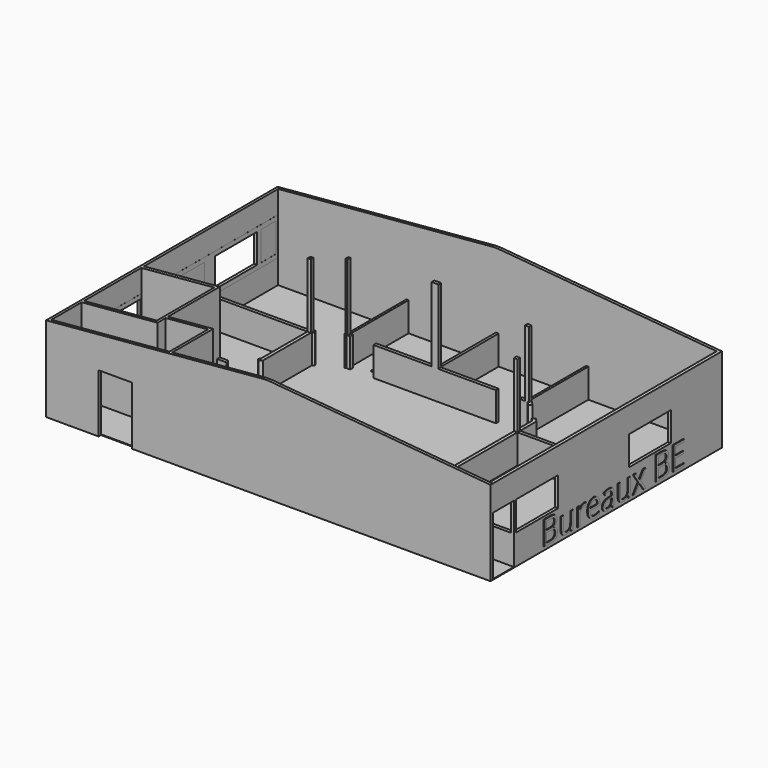
from build123d import *

# Parameters (mm, degrees)
F0_W            = 15040
F0_H            = 9720
F1_DEPTH        = 25
F2_W            = 15240
F2_H            = 9920
F2_W_2          = 100
F2_H_2          = 2105
F3_DEPTH        = 3550
F3_DEPTH_BACK   = 25
F4_W            = 1800
F4_H            = 1000
F5_DEPTH        = 100
F6_W            = 1800
F6_H            = 1000
F7_DEPTH        = 100
F8_W            = 1150
F8_H            = 2000
F9_DEPTH        = 100
F10_W           = 800
F10_H           = 2000
F11_DEPTH       = 100
F13_DEPTH       = 9920.001
F14_W           = 900
F14_H           = 2000
F15_DEPTH       = 100
F16_W           = 115
F16_H           = 115
F16_W_2         = 75
F16_W_3         = 126.4718625761
F16_W_4         = 85
F16_H_2         = 2500
F17_DEPTH       = 2550
F19_DEPTH       = 1
F20_W           = 1150
F20_H           = 1995.2939233818
F21_DEPTH       = 1
F22_W           = 1557.891368866
F22_H           = 1000
F22_W_2         = 1800
F22_W_3         = 1859.8644733429
F23_DEPTH       = 1
F24_W           = 1557.891368866
F24_H           = 1000
F24_W_2         = 1800
F24_W_3         = 1859.8644733429
F25_DEPTH       = 1
F26_W           = 8319
F26_H           = 2928.7534618515
F26_W_2         = 1800
F26_H_2         = 1000
F26_W_3         = 2364.8843765259
F26_W_4         = 644.2222595215
F27_DEPTH       = 1
F28_W           = 8319
F28_H           = 1300
F28_W_2         = 1800
F28_H_2         = 1000
F28_W_3         = 2364.8843765259
F28_W_4         = 644.2222595215
F29_DEPTH       = 1
F30_W           = 1150
F30_H           = 2000
F31_DEPTH       = 1
F32_W           = 800
F32_H           = 115
F33_DEPTH       = 1000
F34_TEXT_SIZE   = 952.5378545125
F34_TEXT_SIZE_2 = 810.1748095618
F35_DEPTH       = 25
F36_TEXT_SIZE   = 1144.444435421
F37_DEPTH       = 25


# Not quite as in the source:
# - Text() gives the source's letters only with a copy of the font that has no kerning and outlines rounded to 1/6400 em; it was checked with that copy


with BuildPart() as f1:
    # F0 (on Top) → F1 (new body)
    with BuildSketch(Plane.XY):
        with Locations((-7520, 4860)):
            Rectangle(F0_W, F0_H)
    extrude(amount=F1_DEPTH)

    # F2 (on face) → F3 (join, two sides)
    with BuildSketch(Plane.XY.offset(25)) as f3_sk:
        with Locations((-7520, 4860)):
            Rectangle(F2_W, F2_H)
        Polygon((-15040, 0), (-15040, 1300), (-15040, 1400), (-15040, 3855), (-15040, 3970), (-15040, 6605), (-15040, 6720), (-15040, 9720), (-10640, 9720), (-10565, 9720), (-7565, 9720), (-7475, 9720), (-4475, 9720), (-4400, 9720), (0, 9720), (0, 5670), (0, 5555), (0, 1015), (0, 900), (0, 0), (-10890, 0), (-10990, 0), align=None, mode=Mode.SUBTRACT)
        Polygon((-15040, 1400), (-15040, 1300), (-12440, 1300), (-12440, 1650), (-10990, 1650), (-10990, 0), (-10890, 0), (-10890, 1750), (-12440, 1750), (-12540, 1750), (-12540, 1400), align=None)
        with Locations((-12490, 2802.5)):
            Rectangle(F2_W_2, F2_H_2)
        Polygon((-15040, 3970), (-15040, 3855), (-12540, 3855), (-12440, 3855), (-12117.9646455628, 3855), (-11425, 4547.9646455628), (-11425, 6652.3336148652), (-10610.2005067573, 7105), (-4396.1626970968, 7105), (-3615, 6323.8373029032), (-3615, 4846.8259293999), (-3615, 2035.0966799188), (-2479.9033200812, 900), (0, 900), (0, 1015), (-2432.2687604083, 1015), (-3500, 2082.7312395917), (-3500, 5555), (0, 5555), (0, 5670), (-3500, 5670), (-3500, 6371.4718625761), (-4348.5281374239, 7220), (-4400, 7220), (-4400, 9720), (-4475, 9720), (-4475, 7220), (-7475, 7220), (-7475, 9720), (-7565, 9720), (-7565, 7220), (-10565, 7220), (-10565, 9720), (-10640, 9720), (-10640, 7220), (-11540, 6720), (-15040, 6720), (-15040, 6605), (-11540, 6605), (-11540, 4595.5992052357), (-12165.5992052357, 3970), align=None)
    extrude(amount=F3_DEPTH)
    extrude(f3_sk.sketch, amount=-F3_DEPTH_BACK)

    # F4 (on face) → F5 (cut, through all)
    with BuildSketch(Plane.YZ.offset(100)):
        with Locations((1900, 1525)):
            Rectangle(F4_W, F4_H)
        with Locations((6730, 1525)):
            Rectangle(F4_W, F4_H)
    extrude(amount=-F5_DEPTH, mode=Mode.SUBTRACT)

    # F6 (on face) → F7 (cut, through all)
    with BuildSketch(Plane(origin=(-15140, 0, 0), x_dir=(0, -1, 0), z_dir=(-1, 0, 0))):
        with Locations((-7920, 1500)):
            Rectangle(F6_W, F6_H)
        with Locations((-2910, 1500)):
            Rectangle(F6_W, F6_H)
    extrude(amount=-F7_DEPTH, mode=Mode.SUBTRACT)

    # F8 (on face) → F9 (cut, through all)
    with BuildSketch(Plane.XZ.offset(100)):
        with Locations((-12765, 1000)):
            Rectangle(F8_W, F8_H)
    extrude(amount=-F9_DEPTH, mode=Mode.SUBTRACT)

    # F10 (on face) → F11 (cut, through all)
    with BuildSketch(Plane.YZ.offset(-10890)):
        with Locations((530, 1025)):
            Rectangle(F10_W, F10_H)
    extrude(amount=-F11_DEPTH, mode=Mode.SUBTRACT)

    # F12 (on face) → F13 (cut, through all)
    with BuildSketch(Plane(origin=(0, 9820, 0), x_dir=(-1, 0, 0), z_dir=(0, 1, 0))):
        Polygon((15140, 3575), (7680, 3575), (15140, 2919.9729382354), align=None)
        Polygon((-100, 2909.436309896), (7480, 3575), (-100, 3575), align=None)
    extrude(amount=-F13_DEPTH, mode=Mode.SUBTRACT)

    # F14 (on face) → F15 (cut, through all)
    with BuildSketch(Plane(origin=(0, 0, 0), x_dir=(0, -1, 0), z_dir=(-1, 0, 0))):
        with Locations((-450, 1025)):
            Rectangle(F14_W, F14_H)
    extrude(amount=-F15_DEPTH, mode=Mode.SUBTRACT)

    # F16 (on face) → F17 (cut)
    with BuildSketch(Plane.XY.offset(3575)):
        Polygon((-7814.558506012, 9720), (-15040, 9720), (-15040, 3970), (-12440, 3970), (-12440, 3855), (-6280.3726196289, 0), (0, 0), (0, 9720), (-7426.3219833374, 9720), (-7480, 9720), (-7480, 7220), (-7450, 7220), (-7450, 7105), (-7480, 7105), (-7565, 7105), (-7680, 7105), (-7680, 7220), (-7565, 7220), (-7565, 9720), (-7680, 9720), align=None)
        with Locations((-11482.5, 6662.5)):
            Rectangle(F16_W, F16_H, mode=Mode.SUBTRACT)
        with Locations((-10602.5, 7162.5)):
            Rectangle(F16_W_2, F16_H, mode=Mode.SUBTRACT)
        with Locations((-4411.7640687119, 7162.5)):
            Rectangle(F16_W_3, F16_H, mode=Mode.SUBTRACT)
        with Locations((-3557.5, 5612.5)):
            Rectangle(F16_W, F16_H, mode=Mode.SUBTRACT)
        with Locations((-7522.5, 8470)):
            Rectangle(F16_W_4, F16_H_2)
    extrude(amount=-F17_DEPTH, mode=Mode.SUBTRACT)

    # F32 (on face) → F33 (cut, through all)
    with BuildSketch(Plane.XY.offset(1025)):
        Polygon((-11587.6345596729, 4547.9646455628), (-12165.5992052357, 3970), (-12084.2819253993, 3888.6827201635), (-11506.3172798365, 4466.6473657264), align=None)
        Polygon((-10712.4843724739, 7179.7309041812), (-11411.8101933712, 6791.2165592382), (-11355.9612562856, 6690.6884724843), (-10656.6354353884, 7079.2028174272), align=None)
        with Locations((-10075.8462905884, 7162.5)):
            Rectangle(F32_W, F32_H)
        with Locations((-5075.8462905884, 7162.5)):
            Rectangle(F32_W, F32_H)
        Polygon((-3619.2766952966, 6490.7485578728), (-4184.9621202459, 7056.433982822), (-4266.2794000823, 6975.1167029856), (-3700.5939751331, 6409.4312780363), align=None)
        Polygon((-2658.253017766, 1240.9842573576), (-3223.9384427152, 1806.6696823069), (-3305.2557225516, 1725.3524024704), (-2739.5702976024, 1159.6669775212), align=None)
    extrude(amount=-F33_DEPTH, mode=Mode.SUBTRACT)

    # F34 (on face) → F35 (join)
    with BuildSketch(Plane.XY.offset(25)):
        with Locations((-14548.2091903687, 2320.752620697)):
            Text('WC', F34_TEXT_SIZE, font='Open Sans', text_align=(TextAlign.LEFT, TextAlign.BOTTOM))
        with Locations((-9903.5501480103, 7513.1554603577)):
            Text('Jean', F34_TEXT_SIZE_2, font='Open Sans', text_align=(TextAlign.LEFT, TextAlign.BOTTOM))
    extrude(amount=F35_DEPTH)

    # F36 (on face) → F37 (join)
    with BuildSketch(Plane.YZ.offset(100)):
        with Locations((2068.0000782013, 121.916718781)):
            Text('Bureaux BE', F36_TEXT_SIZE, font='Open Sans', text_align=(TextAlign.LEFT, TextAlign.BOTTOM))
    extrude(amount=F37_DEPTH)


with BuildPart() as f19:
    # F18 (on face) → F19 (new body)
    with BuildSketch(Plane.XZ.offset(-9720)):
        Polygon((-15040, 2928.7534618515), (-15040, 25), (0, 0), (0, 2918.2168335122), (-7480.0000000002, 3575), (-7679.9999999999, 3575), align=None)
    extrude(amount=F19_DEPTH)


with BuildPart() as f21:
    # F20 (on face) → F21 (new body)
    with BuildSketch(Plane(origin=(0, 0, 0), x_dir=(-1, 0, 0), z_dir=(0, 1, 0))):
        Polygon((7480, 3575), (0, 2918.2168335122), (-100, 2918.2168335122), (-100, 25), (12190, 4.7060766182), (15040, 0), (15040, 2928.7534618515), (7679.9999999999, 3575), align=None)
        with Locations((12765, 1002.3530383091)):
            Rectangle(F20_W, F20_H, mode=Mode.SUBTRACT)
        with Locations((12765, 1002.3530383091)):
            Rectangle(F20_W, F20_H)
    extrude(amount=F21_DEPTH)

    # F30 (on face) → F31 (cut, through all)
    with BuildSketch(Plane.XZ):
        with Locations((-12765, 1000)):
            Rectangle(F30_W, F30_H)
    extrude(amount=-F31_DEPTH, mode=Mode.SUBTRACT)


with BuildPart() as f23:
    # F22 (on face) → F23 (new body)
    with BuildSketch(Plane(origin=(0, 0, 0), x_dir=(0, -1, 0), z_dir=(-1, 0, 0))):
        Polygon((0, 2918.2168335122), (-9720, 2918.2168335122), (-9720, 25), (-5670, 25), (-5670, 1025), (-5555, 1025), (-5555, 25), (-1015, 25), (-1015, 1025), (-2800, 1025), (-2800, 2025), (-999.9999999999, 2025), (-999.9999999999, 1025), (-900, 1025), (-900, 2025), (0, 2025), align=None)
        with Locations((-8649.7595310211, 1525)):
            Rectangle(F22_W, F22_H, mode=Mode.SUBTRACT)
        with Locations((-6730, 1525)):
            Rectangle(F22_W_2, F22_H, mode=Mode.SUBTRACT)
        with Locations((-4386.6227865219, 1525)):
            Rectangle(F22_W_3, F22_H, mode=Mode.SUBTRACT)
    extrude(amount=F23_DEPTH)


with BuildPart() as f25:
    # F24 (on face) → F25 (new body)
    with BuildSketch(Plane(origin=(-1, 0, 0), x_dir=(0, -1, 0), z_dir=(-1, 0, 0))):
        Polygon((0, 2175), (-9720, 2175), (-9720, 875), (-5670, 875), (-5670, 1025), (-5555, 1025), (-5555, 875), (-1015, 875), (-1015, 1025), (-2800, 1025), (-2800, 2025), (-999.9999999999, 2025), (-999.9999999999, 1025), (-900, 1025), (-900, 2025), (0, 2025), align=None)
        with Locations((-8649.7595310211, 1525)):
            Rectangle(F24_W, F24_H, mode=Mode.SUBTRACT)
        with Locations((-6730, 1525)):
            Rectangle(F24_W_2, F24_H, mode=Mode.SUBTRACT)
        with Locations((-4386.6227865219, 1525)):
            Rectangle(F24_W_3, F24_H, mode=Mode.SUBTRACT)
    extrude(amount=F25_DEPTH)


with BuildPart() as f27:
    # F26 (on face) → F27 (new body)
    with BuildSketch(Plane.YZ.offset(-15040)):
        with Locations((5559.5, 1464.3767309258)):
            Rectangle(F26_W, F26_H)
        with Locations((2910, 1500)):
            Rectangle(F26_W_2, F26_H_2, mode=Mode.SUBTRACT)
        with Locations((5388.0257606506, 1500)):
            Rectangle(F26_W_3, F26_H_2, mode=Mode.SUBTRACT)
        with Locations((7920, 1500)):
            Rectangle(F26_W_2, F26_H_2, mode=Mode.SUBTRACT)
        with Locations((9312.370300293, 1500)):
            Rectangle(F26_W_4, F26_H_2, mode=Mode.SUBTRACT)
    extrude(amount=F27_DEPTH)


with BuildPart() as f29:
    # F28 (on face) → F29 (new body)
    with BuildSketch(Plane.YZ.offset(-15039)):
        with Locations((5559.5, 1500)):
            Rectangle(F28_W, F28_H)
        with Locations((2910, 1500)):
            Rectangle(F28_W_2, F28_H_2, mode=Mode.SUBTRACT)
        with Locations((5388.0257606506, 1500)):
            Rectangle(F28_W_3, F28_H_2, mode=Mode.SUBTRACT)
        with Locations((7920, 1500)):
            Rectangle(F28_W_2, F28_H_2, mode=Mode.SUBTRACT)
        with Locations((9312.370300293, 1500)):
            Rectangle(F28_W_4, F28_H_2, mode=Mode.SUBTRACT)
    extrude(amount=F29_DEPTH)


solid = Compound([f1.part, f19.part, f21.part, f23.part, f25.part, f27.part, f29.part])
